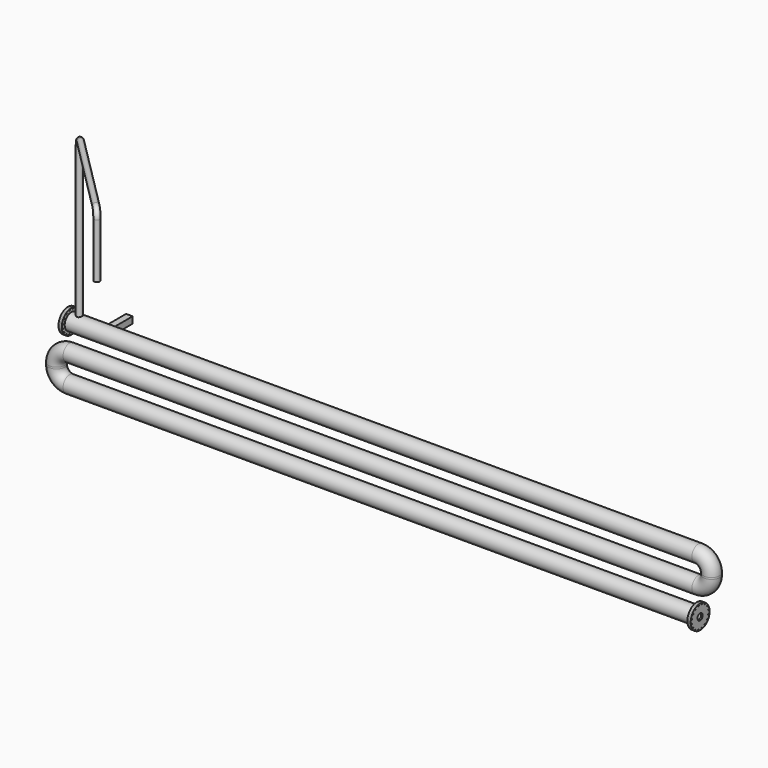
from build123d import *

# Parameters (mm, degrees)
F2_R      = 127
F2_R_2    = 120.65
F5_DEPTH  = 25.4
F10_R     = 44.45
F10_R_2   = 38.9636
F15_DEPTH = 25.4
F17_R     = 184.15
F17_R_2   = 7.9375
F17_R_3   = 127
F18_DEPTH = 25.4
F19_R     = 184.15
F19_R_2   = 7.9375
F19_R_3   = 50.7746
F20_DEPTH = 25.4
F21_R     = 184.15
F21_R_2   = 7.9375
F21_R_3   = 127
F22_DEPTH = 25.4
F23_R     = 184.15
F23_R_2   = 7.9375
F23_R_3   = 50.7746
F24_DEPTH = 25.4
F26_W     = 101.6
F26_H     = 101.6
F27_DEPTH = 25.4
F29_DEPTH = 368.3


# Not quite as in the source:
# - a feature names something its author has since deleted; it is built from what else it names


with BuildPart() as f3:
    # F3: sweep along a path in F0
    with BuildLine(Plane.XZ) as f3_path:
        Line((-4889.5, 431.8), (4889.5, 431.8))
        ThreePointArc((4889.5, 431.8), (5033.1840979371, 372.2840979371), (5092.7, 228.6))
        Line((5092.7, 228.6), (5092.7, 203.2))
        ThreePointArc((5092.7, 203.2), (5033.1840979371, 59.5159020629), (4889.5, 0))
        Line((4889.5, 0), (-4889.5, 0))
        ThreePointArc((-4889.5, 0), (-5033.1840979371, -59.5159020629), (-5092.7, -203.2))
        Line((-5092.7, -203.2), (-5092.7, -228.6))
        ThreePointArc((-5092.7, -228.6), (-5033.1840979371, -372.2840979371), (-4889.5, -431.8))
        Line((-4889.5, -431.8), (4890.804485321, -431.8))
    # F2 (on line) → F3 (sweep)
    with BuildSketch(Plane.YZ.offset(-4889.5)):
        with Locations((0, 431.8)):
            Circle(F2_R)
        with Locations((0, 431.8)):
            Circle(F2_R_2, mode=Mode.SUBTRACT)
    sweep(path=f3_path.line)

    # F2 (on line) → F5 (join)
    with BuildSketch(Plane.YZ.offset(-4889.5)):
        with Locations((0, 431.8)):
            Circle(F2_R)
        with Locations((0, 431.8)):
            Circle(F2_R_2, mode=Mode.SUBTRACT)
        with Locations((0, 431.8)):
            Circle(F2_R_2)
    extrude(amount=F5_DEPTH)

    # F10 (on face) → F15 (join)
    with BuildSketch(Plane(origin=(0, 0, 558.8), x_dir=(1, 0, 0), z_dir=(0, 0, -1))):
        with Locations((-4737.1, 0)):
            Circle(F10_R)
        with Locations((-4737.1, 0)):
            Circle(F10_R_2, mode=Mode.SUBTRACT)
    extrude(amount=F15_DEPTH)

    # F16: sweep along a path in F14
    with BuildLine(Plane(origin=(-2368.55, -2368.55, 0), x_dir=(0.7071067812, -0.7071067812, 0), z_dir=(-0.7071067812, -0.7071067812, 0))) as f16_path:
        Line((-3349.6355331588, 558.8), (-3349.6355331588, 2882.9))
        ThreePointArc((-3349.6355331588, 2882.9), (-3316.1578382484, 2963.7223050896), (-3235.3355331588, 2997.2))
        Line((-3235.3355331588, 2997.2), (-1533.5355331588, 2997.2))
        ThreePointArc((-1533.5355331588, 2997.2), (-1452.7132280692, 2963.7223050896), (-1419.2355331588, 2882.9))
        Line((-1419.2355331588, 2882.9), (-1419.2355331588, 2032))
    # F10 (on face) → F16 (sweep)
    with BuildSketch(Plane(origin=(0, 0, 558.8), x_dir=(1, 0, 0), z_dir=(0, 0, -1))):
        with Locations((-4737.1, 0)):
            Circle(F10_R)
        with Locations((-4737.1, 0)):
            Circle(F10_R_2, mode=Mode.SUBTRACT)
    sweep(path=f16_path.line)

    # F17 (on face) → F18 (join)
    with BuildSketch(Plane.YZ.offset(-4889.5)):
        with Locations((0, 431.8)):
            Circle(F17_R)
        with Locations((-93.4885809614, 291.8844509898)):
            Circle(F17_R_2, mode=Mode.SUBTRACT)
        with Locations((-139.9155490102, 338.3114190386)):
            Circle(F17_R_2, mode=Mode.SUBTRACT)
        with Locations((-32.8288239373, 266.7583569401)):
            Circle(F17_R_2, mode=Mode.SUBTRACT)
        with Locations((-165.0416430599, 398.9711760627)):
            Circle(F17_R_2, mode=Mode.SUBTRACT)
        with Locations((32.8288239373, 266.7583569401)):
            Circle(F17_R_2, mode=Mode.SUBTRACT)
        with Locations((93.4885809614, 291.8844509898)):
            Circle(F17_R_2, mode=Mode.SUBTRACT)
        with Locations((139.9155490102, 338.3114190386)):
            Circle(F17_R_2, mode=Mode.SUBTRACT)
        with Locations((165.0416430599, 398.9711760627)):
            Circle(F17_R_2, mode=Mode.SUBTRACT)
        with Locations((-165.0416430599, 464.6288239373)):
            Circle(F17_R_2, mode=Mode.SUBTRACT)
        with Locations((-139.9155490102, 525.2885809614)):
            Circle(F17_R_2, mode=Mode.SUBTRACT)
        with Locations((-93.4885809614, 571.7155490102)):
            Circle(F17_R_2, mode=Mode.SUBTRACT)
        with Locations((-32.8288239373, 596.8416430599)):
            Circle(F17_R_2, mode=Mode.SUBTRACT)
        with Locations((0, 431.8)):
            Circle(F17_R_3, mode=Mode.SUBTRACT)
        with Locations((165.0416430599, 464.6288239373)):
            Circle(F17_R_2, mode=Mode.SUBTRACT)
        with Locations((32.8288239373, 596.8416430599)):
            Circle(F17_R_2, mode=Mode.SUBTRACT)
        with Locations((139.9155490102, 525.2885809614)):
            Circle(F17_R_2, mode=Mode.SUBTRACT)
        with Locations((93.4885809614, 571.7155490102)):
            Circle(F17_R_2, mode=Mode.SUBTRACT)
    extrude(amount=F18_DEPTH)

    # F19 (on face) → F20 (join)
    with BuildSketch(Plane(origin=(-4889.5, 0, 0), x_dir=(0, -1, 0), z_dir=(-1, 0, 0))):
        with Locations((0, 431.8)):
            Circle(F19_R)
        with Locations((-93.4885809614, 291.8844509898)):
            Circle(F19_R_2, mode=Mode.SUBTRACT)
        with Locations((-139.9155490102, 338.3114190386)):
            Circle(F19_R_2, mode=Mode.SUBTRACT)
        with Locations((-32.8288239373, 266.7583569401)):
            Circle(F19_R_2, mode=Mode.SUBTRACT)
        with Locations((-165.0416430599, 398.9711760627)):
            Circle(F19_R_2, mode=Mode.SUBTRACT)
        with Locations((32.8288239373, 266.7583569401)):
            Circle(F19_R_2, mode=Mode.SUBTRACT)
        with Locations((93.4885809614, 291.8844509898)):
            Circle(F19_R_2, mode=Mode.SUBTRACT)
        with Locations((139.9155490102, 338.3114190386)):
            Circle(F19_R_2, mode=Mode.SUBTRACT)
        with Locations((165.0416430599, 398.9711760627)):
            Circle(F19_R_2, mode=Mode.SUBTRACT)
        with Locations((-165.0416430599, 464.6288239373)):
            Circle(F19_R_2, mode=Mode.SUBTRACT)
        with Locations((-139.9155490102, 525.2885809614)):
            Circle(F19_R_2, mode=Mode.SUBTRACT)
        with Locations((-93.4885809614, 571.7155490102)):
            Circle(F19_R_2, mode=Mode.SUBTRACT)
        with Locations((-32.8288239373, 596.8416430599)):
            Circle(F19_R_2, mode=Mode.SUBTRACT)
        with Locations((0, 431.8)):
            Circle(F19_R_3, mode=Mode.SUBTRACT)
        with Locations((165.0416430599, 464.6288239373)):
            Circle(F19_R_2, mode=Mode.SUBTRACT)
        with Locations((32.8288239373, 596.8416430599)):
            Circle(F19_R_2, mode=Mode.SUBTRACT)
        with Locations((139.9155490102, 525.2885809614)):
            Circle(F19_R_2, mode=Mode.SUBTRACT)
        with Locations((93.4885809614, 571.7155490102)):
            Circle(F19_R_2, mode=Mode.SUBTRACT)
    extrude(amount=F20_DEPTH)

    # F21 (on face) → F22 (join)
    with BuildSketch(Plane.YZ.offset(4890.804485321)):
        with Locations((0, -431.8)):
            Circle(F21_R)
        with Locations((-93.4885809614, -571.7155490102)):
            Circle(F21_R_2, mode=Mode.SUBTRACT)
        with Locations((-139.9155490102, -525.2885809614)):
            Circle(F21_R_2, mode=Mode.SUBTRACT)
        with Locations((-32.8288239373, -596.8416430599)):
            Circle(F21_R_2, mode=Mode.SUBTRACT)
        with Locations((-165.0416430599, -464.6288239373)):
            Circle(F21_R_2, mode=Mode.SUBTRACT)
        with Locations((32.8288239373, -596.8416430599)):
            Circle(F21_R_2, mode=Mode.SUBTRACT)
        with Locations((93.4885809614, -571.7155490102)):
            Circle(F21_R_2, mode=Mode.SUBTRACT)
        with Locations((139.9155490102, -525.2885809614)):
            Circle(F21_R_2, mode=Mode.SUBTRACT)
        with Locations((165.0416430599, -464.6288239373)):
            Circle(F21_R_2, mode=Mode.SUBTRACT)
        with Locations((-165.0416430599, -398.9711760627)):
            Circle(F21_R_2, mode=Mode.SUBTRACT)
        with Locations((-139.9155490102, -338.3114190386)):
            Circle(F21_R_2, mode=Mode.SUBTRACT)
        with Locations((-93.4885809614, -291.8844509898)):
            Circle(F21_R_2, mode=Mode.SUBTRACT)
        with Locations((-32.8288239373, -266.7583569401)):
            Circle(F21_R_2, mode=Mode.SUBTRACT)
        with Locations((0, -431.8)):
            Circle(F21_R_3, mode=Mode.SUBTRACT)
        with Locations((165.0416430599, -398.9711760627)):
            Circle(F21_R_2, mode=Mode.SUBTRACT)
        with Locations((32.8288239373, -266.7583569401)):
            Circle(F21_R_2, mode=Mode.SUBTRACT)
        with Locations((139.9155490102, -338.3114190386)):
            Circle(F21_R_2, mode=Mode.SUBTRACT)
        with Locations((93.4885809614, -291.8844509898)):
            Circle(F21_R_2, mode=Mode.SUBTRACT)
    extrude(amount=-F22_DEPTH)

    # F23 (on face) → F24 (join)
    with BuildSketch(Plane.YZ.offset(4890.804485321)):
        with Locations((0, -431.8)):
            Circle(F23_R)
        with Locations((-93.4885809614, -571.7155490102)):
            Circle(F23_R_2, mode=Mode.SUBTRACT)
        with Locations((-139.9155490102, -525.2885809614)):
            Circle(F23_R_2, mode=Mode.SUBTRACT)
        with Locations((-32.8288239373, -596.8416430599)):
            Circle(F23_R_2, mode=Mode.SUBTRACT)
        with Locations((-165.0416430599, -464.6288239373)):
            Circle(F23_R_2, mode=Mode.SUBTRACT)
        with Locations((32.8288239373, -596.8416430599)):
            Circle(F23_R_2, mode=Mode.SUBTRACT)
        with Locations((93.4885809614, -571.7155490102)):
            Circle(F23_R_2, mode=Mode.SUBTRACT)
        with Locations((139.9155490102, -525.2885809614)):
            Circle(F23_R_2, mode=Mode.SUBTRACT)
        with Locations((165.0416430599, -464.6288239373)):
            Circle(F23_R_2, mode=Mode.SUBTRACT)
        with Locations((-165.0416430599, -398.9711760627)):
            Circle(F23_R_2, mode=Mode.SUBTRACT)
        with Locations((-139.9155490102, -338.3114190386)):
            Circle(F23_R_2, mode=Mode.SUBTRACT)
        with Locations((-93.4885809614, -291.8844509898)):
            Circle(F23_R_2, mode=Mode.SUBTRACT)
        with Locations((-32.8288239373, -266.7583569401)):
            Circle(F23_R_2, mode=Mode.SUBTRACT)
        with Locations((0, -431.8)):
            Circle(F23_R_3, mode=Mode.SUBTRACT)
        with Locations((165.0416430599, -398.9711760627)):
            Circle(F23_R_2, mode=Mode.SUBTRACT)
        with Locations((32.8288239373, -266.7583569401)):
            Circle(F23_R_2, mode=Mode.SUBTRACT)
        with Locations((139.9155490102, -338.3114190386)):
            Circle(F23_R_2, mode=Mode.SUBTRACT)
        with Locations((93.4885809614, -291.8844509898)):
            Circle(F23_R_2, mode=Mode.SUBTRACT)
    extrude(amount=F24_DEPTH)

    # F26 (on face) → F27 (join)
    with BuildSketch(Plane(origin=(0, 127, 0), x_dir=(-1, 0, 0), z_dir=(0, 1, 0))):
        with Locations((4356.1, 431.8)):
            Rectangle(F26_W, F26_H)
    extrude(amount=-F27_DEPTH)

    # F28 (on face) → F29 (join, through all)
    with BuildSketch(Plane.XZ.offset(-495.3)):
        Polygon((-4406.9, 431.8), (-4406.9, 381), (-4305.3, 381), (-4305.3, 431.8), (-4305.3, 482.6), (-4406.9, 482.6), align=None)
    extrude(amount=F29_DEPTH)


solid = f3.part
